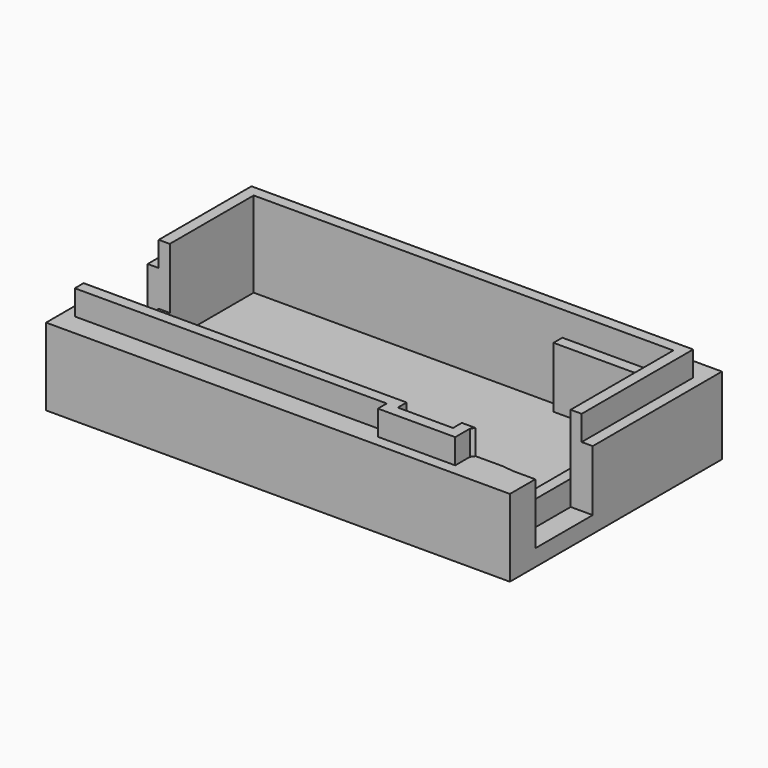
from build123d import *

# Parameters (mm, degrees)
F0_W     = 2
F0_H     = 19
F0_H_2   = 16
F0_W_2   = 18.0994240791
F0_H_3   = 2
F0_H_4   = 1
F0_H_5   = 23.25
F0_H_6   = 13
F0_H_7   = 6
F0_W_3   = 10
F0_H_8   = 5.75
F1_DEPTH = 3
F2_DEPTH = 4.5
F3_DEPTH = 11
F5_DEPTH = 4.5
F6_DEPTH = 4.5
F7_DEPTH = 4.5


# Not quite as in the source:
# - a feature names something its author has since deleted; it is built from what else it names


with BuildPart() as f1:
    # F0 (on Top) → F1 (new body)
    with BuildSketch(Plane.XY):
        Polygon((-48.8793104887, -18.5732776225), (-48.8793104887, 0.4267223775), (-46.8793104887, 0.4267223775), (9.0212654322, 0.4267223775), (27.1206895113, 0.4267223775), (29.1206895113, 0.4267223775), (29.1206895113, 6.4267223775), (-50.8793104887, 6.4267223775), (-50.8793104887, -1.5732776225), (-50.8793104887, -18.5732776225), align=None)
        with Locations((-47.8793104887, -9.0732776225)):
            Rectangle(F0_W, F0_H)
        Polygon((9.0212654322, 0.4267223775), (-46.8793104887, 0.4267223775), (-46.8793104887, -18.5732776225), (-46.8793104887, -34.5732776225), (-46.8793104887, -35.5732776225), (9.6206895113, -35.5732776225), (19.6206895113, -35.5732776225), (27.1206895113, -35.5732776225), (27.1206895113, -1.5732776225), (9.0212654322, -1.5732776225), align=None)
        with Locations((-47.8793104887, -26.5732776225)):
            Rectangle(F0_W, F0_H_2)
        with Locations((18.0709774718, -0.5732776225)):
            Rectangle(F0_W_2, F0_H_3)
        with Locations((-47.8793104887, -35.0732776225)):
            Rectangle(F0_W, F0_H_4)
        Polygon((-48.8793104887, -35.5732776225), (-48.8793104887, -34.5732776225), (-50.8793104887, -34.5732776225), (-50.8793104887, -35.5732776225), (-50.8793104887, -41.5732776225), (27.1206895113, -41.5732776225), (27.1206895113, -35.5732776225), (19.6206895113, -35.5732776225), (19.6206895113, -37.5732776225), (9.6206895113, -37.5732776225), (9.6206895113, -35.5732776225), (-46.8793104887, -35.5732776225), align=None)
        Polygon((29.1206895113, 0.4267223775), (27.1206895113, 0.4267223775), (27.1206895113, -1.5732776225), (27.1206895113, -35.5732776225), (29.1206895113, -35.8232776225), (29.1206895113, -22.8232776225), align=None)
        with Locations((30.1206895113, -11.1982776225)):
            Rectangle(F0_W, F0_H_5)
        Polygon((29.1206895113, 6.4267223775), (29.1206895113, 0.4267223775), (31.1206895113, 0.4267223775), (31.1206895113, 6.4267223775), (30.1206895113, 6.4267223775), align=None)
        with Locations((30.1206895113, -29.3232776225)):
            Rectangle(F0_W, F0_H_6)
        with Locations((32.1206895113, -11.1982776225)):
            Rectangle(F0_W, F0_H_5)
        with Locations((32.1206895113, 3.4267223775)):
            Rectangle(F0_W, F0_H_7)
        Polygon((29.1206895113, -35.8232776225), (27.1206895113, -35.5732776225), (27.1206895113, -41.5732776225), (29.1206895113, -41.5732776225), align=None)
        with Locations((14.6206895113, -36.5732776225)):
            Rectangle(F0_W_3, F0_H_3)
        Polygon((31.1206895113, -35.8232776225), (29.1206895113, -35.8232776225), (29.1206895113, -41.5732776225), (30.1206895113, -41.5732776225), (31.1206895113, -41.5732776225), align=None)
        with Locations((32.1206895113, -29.3232776225)):
            Rectangle(F0_W, F0_H_6)
        with Locations((32.1206895113, -38.6982776225)):
            Rectangle(F0_W, F0_H_8)
    extrude(amount=-F1_DEPTH)

    # F0 (on Top) → F2 (join)
    with BuildSketch(Plane.XY):
        with Locations((-47.8793104887, -9.0732776225)):
            Rectangle(F0_W, F0_H)
        with Locations((-47.8793104887, -26.5732776225)):
            Rectangle(F0_W, F0_H_2)
        with Locations((18.0709774718, -0.5732776225)):
            Rectangle(F0_W_2, F0_H_3)
        with Locations((-47.8793104887, -35.0732776225)):
            Rectangle(F0_W, F0_H_4)
    extrude(amount=F2_DEPTH)

    # F0 (on Top) → F3 (join)
    with BuildSketch(Plane.XY):
        Polygon((-48.8793104887, -18.5732776225), (-48.8793104887, 0.4267223775), (-46.8793104887, 0.4267223775), (9.0212654322, 0.4267223775), (27.1206895113, 0.4267223775), (29.1206895113, 0.4267223775), (29.1206895113, 6.4267223775), (-50.8793104887, 6.4267223775), (-50.8793104887, -1.5732776225), (-50.8793104887, -18.5732776225), align=None)
        with Locations((-47.8793104887, -9.0732776225)):
            Rectangle(F0_W, F0_H)
        with Locations((18.0709774718, -0.5732776225)):
            Rectangle(F0_W_2, F0_H_3)
        Polygon((-48.8793104887, -35.5732776225), (-48.8793104887, -34.5732776225), (-50.8793104887, -34.5732776225), (-50.8793104887, -35.5732776225), (-50.8793104887, -41.5732776225), (27.1206895113, -41.5732776225), (27.1206895113, -35.5732776225), (19.6206895113, -35.5732776225), (19.6206895113, -37.5732776225), (9.6206895113, -37.5732776225), (9.6206895113, -35.5732776225), (-46.8793104887, -35.5732776225), align=None)
        with Locations((30.1206895113, -11.1982776225)):
            Rectangle(F0_W, F0_H_5)
        Polygon((29.1206895113, 6.4267223775), (29.1206895113, 0.4267223775), (31.1206895113, 0.4267223775), (31.1206895113, 6.4267223775), (30.1206895113, 6.4267223775), align=None)
        with Locations((32.1206895113, -11.1982776225)):
            Rectangle(F0_W, F0_H_5)
        with Locations((32.1206895113, 3.4267223775)):
            Rectangle(F0_W, F0_H_7)
        Polygon((29.1206895113, -35.8232776225), (27.1206895113, -35.5732776225), (27.1206895113, -41.5732776225), (29.1206895113, -41.5732776225), align=None)
        Polygon((31.1206895113, -35.8232776225), (29.1206895113, -35.8232776225), (29.1206895113, -41.5732776225), (30.1206895113, -41.5732776225), (31.1206895113, -41.5732776225), align=None)
        with Locations((32.1206895113, -38.6982776225)):
            Rectangle(F0_W, F0_H_8)
    extrude(amount=F3_DEPTH)

    # F4 (on face) → F5 (join)
    with BuildSketch(Plane.XY.offset(11)):
        Polygon((22.1148194903, -35.5732776225), (19.6206895113, -35.5732776225), (19.6206895113, -37.5732776225), (9.6206895113, -37.5732776225), (9.6206895113, -35.5732776225), (-48.8793104887, -35.5732776225), (-48.8793104887, -37.5732776225), (7.6206895113, -37.5732776225), (7.6206895113, -39.5732776225), (21.6206895113, -39.5732776225), (21.6206895113, -36.236452068), align=None)
    extrude(amount=F5_DEPTH)

    # F0 (on Top) → F6 (join)
    with BuildSketch(Plane.XY):
        Polygon((29.1206895113, 0.4267223775), (27.1206895113, 0.4267223775), (27.1206895113, -1.5732776225), (27.1206895113, -35.5732776225), (29.1206895113, -35.8232776225), (29.1206895113, -22.8232776225), align=None)
    extrude(amount=F6_DEPTH)

    # F4 (on face) → F7 (join)
    with BuildSketch(Plane.XY.offset(11)):
        Polygon((31.1206895113, -22.8232776225), (31.1206895113, 2.4267223775), (29.1206895113, 2.4267223775), (-48.8793104887, 2.4267223775), (-48.8793104887, -18.5732776225), (-46.8793104887, -18.5732776225), (-46.8793104887, 0.4267223775), (29.1206895113, 0.4267223775), (29.1206895113, -22.8232776225), align=None)
    extrude(amount=F7_DEPTH)


solid = f1.part
